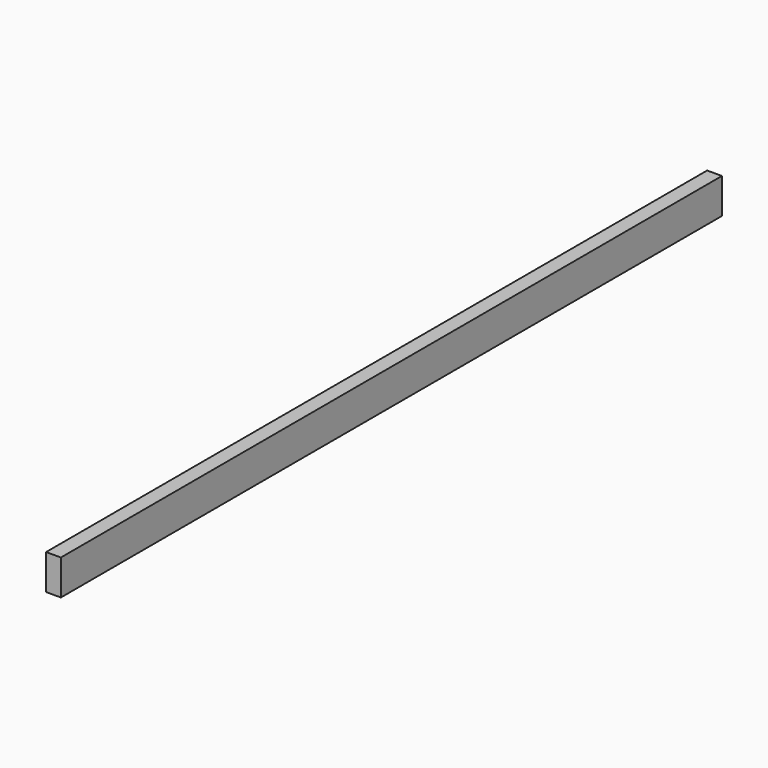
from build123d import *

# Parameters (mm, degrees)
F1_W     = 21
F1_H     = 50
F2_DEPTH = 1173


with BuildPart() as f2:
    # F1 (on Front) → F2 (new body)
    with BuildSketch(Plane.XZ):
        with Locations((10.5, 25)):
            Rectangle(F1_W, F1_H)
    extrude(amount=F2_DEPTH)


solid = f2.part
